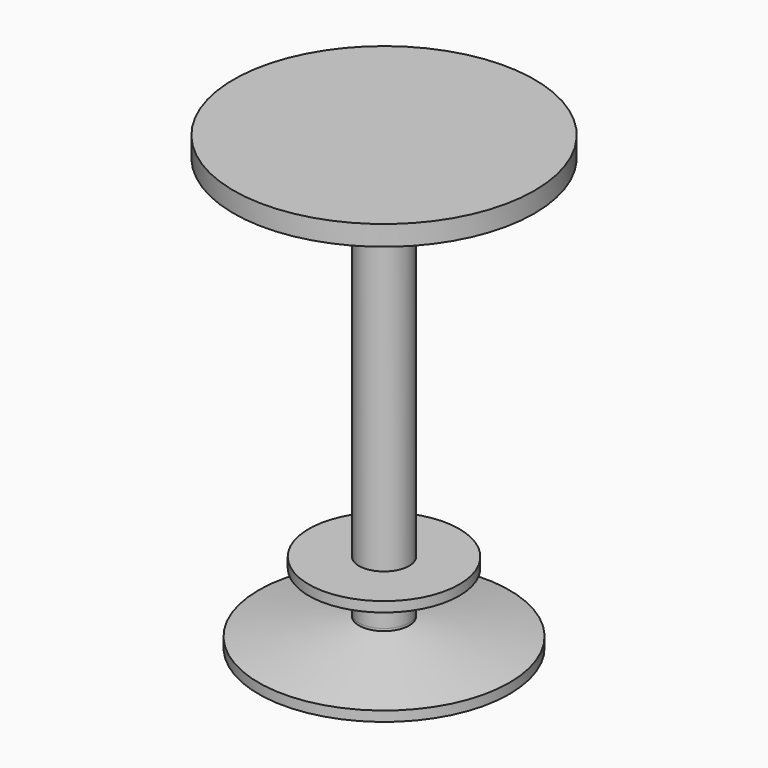
from build123d import *

# Parameters (mm, degrees)
F0_R         = 19.05
F1_DEPTH     = 2.54
F2_R         = 3.175
F3_DEPTH     = 44.45
F4_R         = 9.525
F5_DEPTH     = 1.27
F6_R         = 3.175
F7_DEPTH     = 5.08
F8_R         = 15.875
F9_DEPTH     = 3.81
F10_S5_R     = 3.175
F10_T6_DEPTH = 24


# Not quite as in the source:
# - a fillet or chamfer that OpenCascade refuses, or shapes differently, is made with other operations: its cross-section is extruded or revolved along the edge and cut away or added


with BuildPart() as f1:
    # F0 (on Top) → F1 (new body)
    with BuildSketch(Plane.XY):
        Circle(F0_R)
    extrude(amount=F1_DEPTH)

    # F2 (on face) → F3 (join)
    with BuildSketch(Plane(origin=(0, 0, 0), x_dir=(1, 0, 0), z_dir=(0, 0, -1))):
        Circle(F2_R)
    extrude(amount=F3_DEPTH)

    # F4 (on face) → F5 (join)
    with BuildSketch(Plane(origin=(0, 0, -44.45), x_dir=(1, 0, 0), z_dir=(0, 0, -1))):
        Circle(F4_R)
    extrude(amount=F5_DEPTH)

    # F6 (on face) → F7 (join)
    with BuildSketch(Plane(origin=(0, 0, -45.72), x_dir=(1, 0, 0), z_dir=(0, 0, -1))):
        Circle(F6_R)
    extrude(amount=F7_DEPTH)

    # F8 (on face) → F9 (join)
    with BuildSketch(Plane(origin=(0, 0, -50.8), x_dir=(1, 0, 0), z_dir=(0, 0, -1))):
        Circle(F8_R)
    extrude(amount=F9_DEPTH)

    # F10: chamfer of 2.54 x 14.4050558218 on 1 edges, made by hand


with BuildPart() as f10_tool2:
    # F10_s3 → F10_t4 (revolve)
    with BuildSketch(Plane.XZ):
        Polygon((15.875, -53.34), (1.4699441782, -50.8), (15.875, -50.8), align=None)
    revolve(axis=Axis((0, 0, -50.8), (0, 0, -1)))

    # F10_s5 → F10_t6 (cut, symmetric)
    with BuildSketch(Plane.XY.offset(-52.1)):
        Circle(F10_S5_R)
    extrude(amount=F10_T6_DEPTH, both=True, mode=Mode.SUBTRACT)


with BuildPart() as f1_1:
    add(f1.part)

    # F10_t1: cut F10_tool2
    add(f10_tool2.part, mode=Mode.SUBTRACT)


solid = f1_1.part
